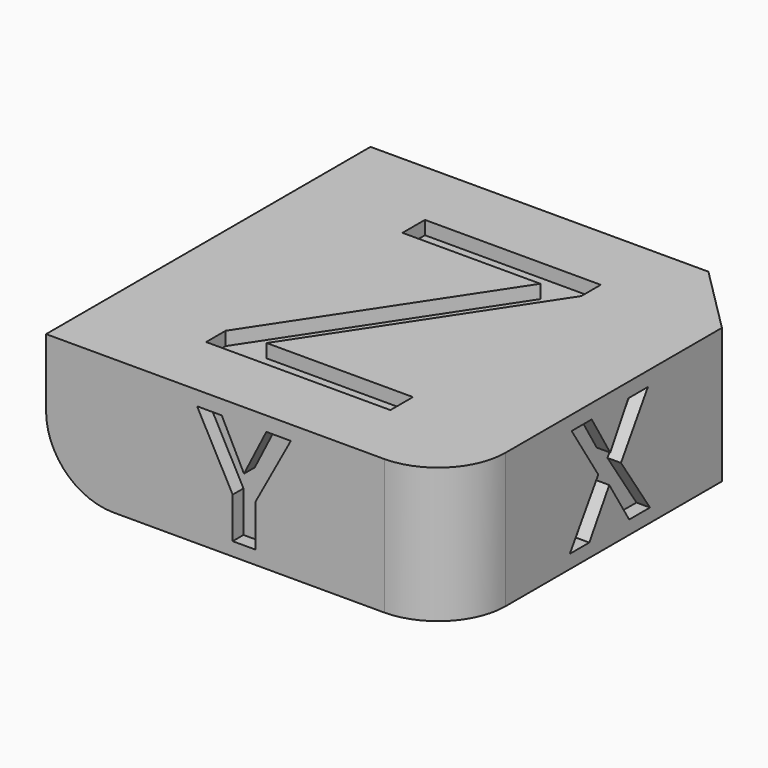
from build123d import *

# Parameters (mm, degrees)
F0_W          = 30
F0_H          = 30
F1_DEPTH      = 10
F3_SIZE       = 5
F4_T1_DEPTH   = 54.999500005
F4_T3_DEPTH   = 34.999500005
F5_TEXT_SIZE  = 11.1111111111
F6_DEPTH      = 1
F7_TEXT_SIZE  = 11.1111111111
F8_DEPTH      = 1
F9_TEXT_SIZE  = 11.1111111111
F10_DEPTH     = 1
F11_W         = 2.9131944444
F11_H         = 1.3559027778
F12_DEPTH     = 2
F13_W         = 5.0903163684
F13_H         = 2.0616319444
F13_W_2       = 1.5676697427
F14_DEPTH     = 1
F15_TEXT_SIZE = 27.7777777778
F16_DEPTH     = 1


# Not quite as in the source:
# - a fillet or chamfer that OpenCascade refuses, or shapes differently, is made with other operations: its cross-section is extruded or revolved along the edge and cut away or added
# - a feature of the source that left no trace in its solid (it failed there, or was rolled back) is left out
# - Text() gives the source's letters only with a copy of the font that has no kerning and outlines rounded to 1/6400 em; it was checked with that copy


with BuildPart() as f1:
    # F0 (on Top) → F1 (new body)
    with BuildSketch(Plane.XY):
        Rectangle(F0_W, F0_H)
    extrude(amount=F1_DEPTH)

    # F3
    f3_edges = [f1.edges().sort_by_distance(p)[0] for p in [
        (15, 15, 5),
    ]]
    chamfer(f3_edges, length=F3_SIZE)

    # F4: fillet of radius 5 on 2 edges, made by hand

    # F4_s2 → F4_t1 (cut)
    with BuildSketch(Plane.XZ.offset(-27.4997500025)):
        with BuildLine():
            ThreePointArc((-10.0001, -0.0001), (-13.5356339059, 1.4643660941), (-15.0001, 4.9999))
            Line((-15.0001, 4.9999), (-15.1001, 4.9999))
            ThreePointArc((-15.1001, 4.9999), (-15.1, 2.49995), (-15.1, 0))
            Line((-15.1, 0), (-15, -0.1))
            ThreePointArc((-15, -0.1), (-12.50005, -0.1), (-10.0001, -0.1001))
            Line((-10.0001, -0.1001), (-10.0001, -0.0001))
        make_face()
    extrude(amount=F4_T1_DEPTH, mode=Mode.SUBTRACT)

    # F4_s4 → F4_t3 (cut)
    with BuildSketch(Plane.XY.offset(-12.4997500025)):
        with BuildLine():
            ThreePointArc((15.0001, -10.0001), (13.5356339059, -13.5356339059), (10.0001, -15.0001))
            Line((10.0001, -15.0001), (10.0001, -15.1001))
            ThreePointArc((10.0001, -15.1001), (12.50005, -15.1), (15, -15.1))
            Line((15, -15.1), (15.1, -15))
            ThreePointArc((15.1, -15), (15.1, -12.50005), (15.1001, -10.0001))
            Line((15.1001, -10.0001), (15.0001, -10.0001))
        make_face()
    extrude(amount=F4_T3_DEPTH, mode=Mode.SUBTRACT)

    # F5 (on face) → F6 (cut)
    with BuildSketch(Plane.XZ.offset(15)):
        with Locations((-3.8272569444, 1)):
            Text('Y', F5_TEXT_SIZE, font='Open Sans', font_style=FontStyle.BOLD, text_align=(TextAlign.LEFT, TextAlign.BOTTOM))
    extrude(amount=-F6_DEPTH, mode=Mode.SUBTRACT)

    # F7 (on face) → F8 (cut)
    with BuildSketch(Plane.YZ.offset(15)):
        with Locations((-4.0659722222, 1)):
            Text('X', F7_TEXT_SIZE, font='Open Sans', font_style=FontStyle.BOLD, text_align=(TextAlign.LEFT, TextAlign.BOTTOM))
    extrude(amount=-F8_DEPTH, mode=Mode.SUBTRACT)

    # F9 (on face) → F10 (cut)
    with BuildSketch(Plane(origin=(0, 15, 0), x_dir=(-1, 0, 0), z_dir=(0, 1, 0))):
        with Locations((-5.6145833333, 1)):
            Text('-Y', F9_TEXT_SIZE, font='Open Sans', font_style=FontStyle.BOLD, text_align=(TextAlign.LEFT, TextAlign.BOTTOM))
    extrude(amount=-F10_DEPTH, mode=Mode.SUBTRACT)

    # F11 (on face) → F12 (cut)
    with BuildSketch(Plane(origin=(-15, 0, 0), x_dir=(0, -1, 0), z_dir=(-1, 0, 0))):
        Polygon((0.2747958095, 4.9682773816), (2.4723607947, 4.9682773816), (2.4522569444, 4.9982638889), (4.9418402778, 8.9322916667), (3.1310763889, 8.9322916667), (1.4539930556, 6.078125), (-0.2543402778, 8.9322916667), (-2.1102430556, 8.9322916667), (0.3532986111, 5.0902777778), align=None)
        Polygon((3.2126736111, 1), (5.1328125, 1), (2.4723607947, 4.9682773816), (0.2747958095, 4.9682773816), (-2.2786458333, 1), (-0.4765625, 1), (1.3671875, 4), align=None)
        with Locations((-4.0651041667, 3.9782986111)):
            Rectangle(F11_W, F11_H)
    extrude(amount=-F12_DEPTH, mode=Mode.SUBTRACT)

    # F13 (on face) → F14 (cut)
    with BuildSketch(Plane(origin=(0, 0, 0), x_dir=(1, 0, 0), z_dir=(0, 0, -1))):
        Polygon((-2.6931423611, -10), (10.9396701389, -10), (10.9396701389, -7.9123263889), (0.1150173611, -7.9123263889), (10.6401909722, 8.0251736111), (10.6401909722, 9.8307291667), (-2.3676215278, 9.8307291667), (-2.3676215278, 7.7560763889), (7.83203125, 7.7560763889), (-2.6931423611, -8.1944444444), align=None)
        with Locations((-7.4865644342, -2.5542534722)):
            Rectangle(F13_W, F13_H)
        with Locations((-10.8155574897, -2.5542534722)):
            Rectangle(F13_W_2, F13_H)
    extrude(amount=-F14_DEPTH, mode=Mode.SUBTRACT)

    # F15 (on face) → F16 (cut)
    with BuildSketch(Plane.XY.offset(10)):
        with Locations((-8.2725694444, -10)):
            Text('Z', F15_TEXT_SIZE, font='Open Sans', text_align=(TextAlign.LEFT, TextAlign.BOTTOM))
    extrude(amount=-F16_DEPTH, mode=Mode.SUBTRACT)


solid = f1.part
